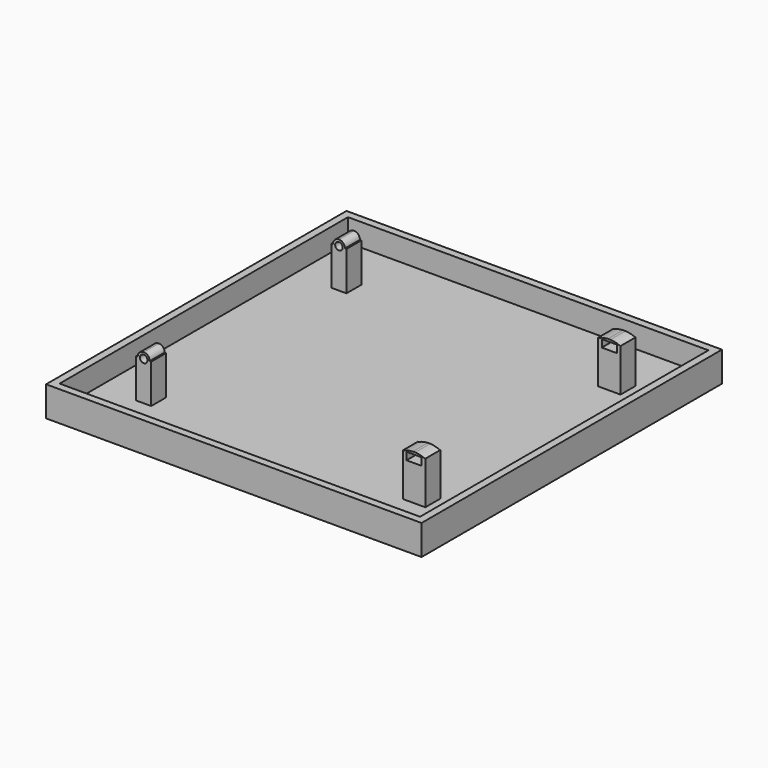
from build123d import *

# Parameters (mm, degrees)
F0_W     = 127
F0_H     = 127
F1_DEPTH = 2.54
F2_W     = 127
F2_H     = 127
F2_W_2   = 121.92
F2_H_2   = 121.92
F3_DEPTH = 7.62
F4_W     = 5.08
F4_H     = 6.35
F4_W_2   = 7.62
F5_DEPTH = 15.24
F6_R     = 1.27
F6_W     = 5.08
F6_H     = 2.54
F7_DEPTH = 6.35


# Not quite as in the source:
# - a pattern or mirror of a feature is missing from the dataset's text; its kind, count and spacing are read off the source's solid


with BuildPart() as f1:
    # F0 (on Top) → F1 (new body)
    with BuildSketch(Plane.XY):
        Rectangle(F0_W, F0_H)
    extrude(amount=F1_DEPTH)

    # F2 (on face) → F3 (join)
    with BuildSketch(Plane.XY.offset(2.54)):
        Rectangle(F2_W, F2_H)
        Rectangle(F2_W_2, F2_H_2, mode=Mode.SUBTRACT)
    extrude(amount=F3_DEPTH)

    # F4 (on face) → F5 (join)
    with BuildSketch(Plane.XY.offset(2.54)):
        with Locations((-45.72, -41.275)):
            Rectangle(F4_W, F4_H)
        with Locations((45.72, -41.275)):
            Rectangle(F4_W_2, F4_H)
    f5 = extrude(amount=F5_DEPTH)

    # F5_copies: F5 across plane
    add(f5.mirror(Plane.ZX))

    # F6 (on face) → F7 (cut)
    with BuildSketch(Plane.XZ.offset(44.45)):
        with Locations((-45.72, 15.748)):
            Circle(F6_R)
        with Locations((45.72, 15.748)):
            Rectangle(F6_W, F6_H)
        with BuildLine():
            Line((-43.18, 17.78), (-45.72, 17.78))
            ThreePointArc((-45.72, 17.78), (-44.2831590206, 17.1848409794), (-43.688, 15.748))
            Line((-43.688, 15.748), (-43.18, 15.748))
            Line((-43.18, 15.748), (-43.18, 17.78))
        make_face()
        with BuildLine():
            ThreePointArc((-47.752, 15.748), (-47.1568409794, 17.1848409794), (-45.72, 17.78))
            Line((-45.72, 17.78), (-48.26, 17.78))
            Line((-48.26, 17.78), (-48.26, 15.748))
            Line((-48.26, 15.748), (-47.752, 15.748))
        make_face()
        with BuildLine():
            Line((49.7070066631, 17.7892204374), (45.72, 17.7892204374))
            ThreePointArc((45.72, 17.7892204374), (47.5717330447, 17.5942784861), (49.3422755435, 17.018))
            Line((49.3422755435, 17.018), (49.7070066631, 17.018))
            Line((49.7070066631, 17.018), (49.7070066631, 17.7892204374))
        make_face()
        with BuildLine():
            ThreePointArc((42.0977244565, 17.018), (43.8682669553, 17.5942784861), (45.72, 17.7892204374))
            Line((45.72, 17.7892204374), (41.827224195, 17.7892204374))
            Line((41.827224195, 17.7892204374), (41.827224195, 17.018))
            Line((41.827224195, 17.018), (42.0977244565, 17.018))
        make_face()
    f7 = extrude(amount=-F7_DEPTH, mode=Mode.SUBTRACT)

    # F7_copies: F7 across plane
    add(f7.mirror(Plane.ZX), mode=Mode.SUBTRACT)


solid = f1.part
